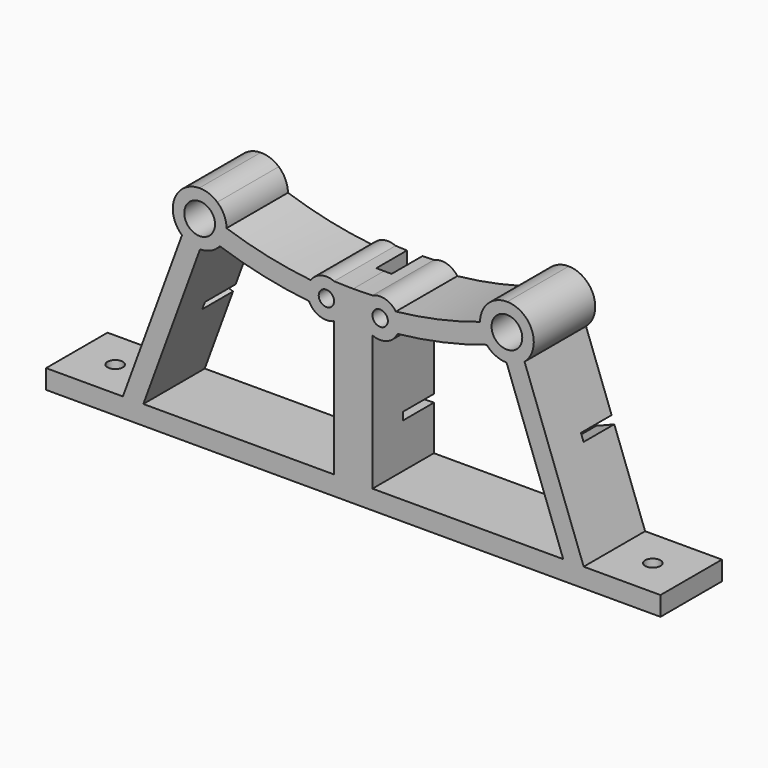
from build123d import *

# Parameters (mm, degrees)
F1_W      = 80
F1_H      = 5
F2_DEPTH  = 10
F3_W      = 5
F3_H      = 151.5
F4_DEPTH  = 10
F5_W      = 21
F5_H      = 23
F6_DEPTH  = 10
F8_DEPTH  = 10
F10_DEPTH = 10
F12_DEPTH = 10
F14_DEPTH = 20
F15_W     = 0.9078182304
F15_H     = 2
F16_DEPTH = 10
F17_R     = 135
F17_R_2   = 133
F18_DEPTH = 10
F19_R     = 7
F19_R_2   = 4
F20_DEPTH = 20
F21_R     = 4
F22_DEPTH = 20.001
F23_R     = 5
F23_R_2   = 2
F24_DEPTH = 20
F26_DEPTH = 20
F28_DEPTH = 20.001
F29_R     = 2
F30_DEPTH = 5.001


# Not quite as in the source:
# - ends of sketch curves that miss each other by under 0.0002 mm in the source are joined


with BuildPart() as f2:
    # F1 (on Front) → F2 (new body)
    with BuildSketch(Plane.XZ):
        with Locations((40, 2.5)):
            Rectangle(F1_W, F1_H)
    extrude(amount=F2_DEPTH)

    # F3 (on Front) → F4 (join, through all)
    with BuildSketch(Plane.XZ):
        with Locations((2.5, 75.75)):
            Rectangle(F3_W, F3_H)
    extrude(amount=F4_DEPTH)

    # F5 (on Front) → F6 (join, through all)
    with BuildSketch(Plane.XZ):
        with Locations((10.5, 151.5)):
            Rectangle(F5_W, F5_H)
    extrude(amount=F6_DEPTH)

    # F7 (on Front) → F8 (join, through all)
    with BuildSketch(Plane.XZ):
        Polygon((60, 5), (9.8688664765, 141.7212732458), (5.1744848971, 140), (55.3056184206, 3.2787267542), align=None)
    extrude(amount=F8_DEPTH)

    # F9 (on face) → F10 (join)
    with BuildSketch(Plane.XZ.offset(10)):
        Polygon((0, 163), (0, 0), (80, 0), (80, 5), (60, 5), (10.5, 140), (21, 140), (21, 163), align=None)
        Polygon((5.1744848971, 140), (54.6744848971, 5), (5, 5), (5, 140), align=None, mode=Mode.SUBTRACT)
    extrude(amount=F10_DEPTH)

    # F11 (on face) → F12 (cut)
    with BuildSketch(Plane(origin=(0, 0, 0), x_dir=(-1, 0, 0), z_dir=(0, 1, 0))):
        Polygon((-2, 0), (0, 0), (0, 140), (-21, 140), (-21, 138), (-2, 138), align=None)
    extrude(amount=-F12_DEPTH, mode=Mode.SUBTRACT)

    # F13 (on face) → F14 (join)
    with BuildSketch(Plane(origin=(0, 0, 0), x_dir=(-1, 0, 0), z_dir=(0, 1, 0))):
        Polygon((-2, 133), (-2, 138), (-11.2333333333, 138), (-13.0666666667, 133), align=None)
    extrude(amount=-F14_DEPTH)

    # F15 (on face) → F16 (join)
    with BuildSketch(Plane.XZ.offset(20)):
        with Locations((5.4539091152, 139)):
            Rectangle(F15_W, F15_H)
    extrude(amount=-F16_DEPTH)

    # F17 (on Front) → F18 (cut)
    with BuildSketch(Plane.XZ):
        with Locations((0, 151.5)):
            Circle(F17_R)
        with Locations((0, 151.5)):
            Circle(F17_R_2, mode=Mode.SUBTRACT)
    extrude(amount=F18_DEPTH, mode=Mode.SUBTRACT)

    # F19 (on Front) → F20 (join, through all)
    with BuildSketch(Plane.XZ):
        with Locations((40.0081513066, 52.2611576598)):
            Circle(F19_R)
        with Locations((40.0081513066, 52.2611576598)):
            Circle(F19_R_2, mode=Mode.SUBTRACT)
    extrude(amount=F20_DEPTH)

    # F21 (on Front) → F22 (cut, through all)
    with BuildSketch(Plane.XZ):
        with Locations((40.0081513066, 52.2611576598)):
            Circle(F21_R)
    extrude(amount=F22_DEPTH, mode=Mode.SUBTRACT)

    # F23 (on Front) → F24 (join, through all)
    with BuildSketch(Plane.XZ):
        with Locations((7, 44.7292174797)):
            Circle(F23_R)
        with Locations((7, 44.7292174797)):
            Circle(F23_R_2, mode=Mode.SUBTRACT)
    extrude(amount=F24_DEPTH)

    # F25 (on Front) → F26 (join, through all)
    with BuildSketch(Plane.XZ):
        with BuildLine():
            Line((8.7843409429, 47.3698633718), (8.9944926401, 44.8787117779))
            ThreePointArc((8.9944926401, 44.8787117779), (22.8274604253, 46.9633698145), (36.2703225327, 50.8348933176))
            Line((36.2703225327, 50.8348933176), (35.4228850903, 53.1868817915))
            ThreePointArc((35.4228850903, 53.1868817915), (22.294150224, 49.4058235462), (8.7843409429, 47.3698633718))
        make_face()
        with BuildLine():
            ThreePointArc((36.2703225327, 50.8348933176), (22.8274604253, 46.9633698145), (8.9944055882, 44.8787044343))
            Line((8.9944055882, 44.8787044343), (9.2046443373, 42.3875601839))
            ThreePointArc((9.2046443373, 42.3875601839), (23.3608559764, 44.5209347206), (37.117759975, 48.4829048437))
            Line((37.117759975, 48.4829048437), (36.2703225327, 50.8348933176))
        make_face()
    extrude(amount=F26_DEPTH)

    # F27 (on Front) → F28 (cut, through all)
    with BuildSketch(Plane.XZ):
        with BuildLine():
            ThreePointArc((5, 49.3117931746), (8.3573933592, 49.5414397593), (11.0998968806, 47.5911828128))
            ThreePointArc((11.0998968806, 47.5911828128), (22.1823046987, 49.3814641789), (33.0087181874, 52.3502419386))
            ThreePointArc((33.0087181874, 52.3502419386), (38.6064619078, 59.1193838757), (46.4113234148, 55.0894764101))
            ThreePointArc((46.4113234148, 55.0894764101), (104.3190443402, 175.3020374745), (0, 258.5))
            Line((0, 258.5), (0, 253.8104570129))
            ThreePointArc((0, 253.8104570129), (-102.2798898997, 148.9992528562), (5, 49.3117931746))
        make_face()
    extrude(amount=F28_DEPTH, mode=Mode.SUBTRACT)

    # F29 (on face) → F30 (cut, through all)
    with BuildSketch(Plane.XY.offset(5)):
        with Locations((70, -10)):
            Circle(F29_R)
    extrude(amount=-F30_DEPTH, mode=Mode.SUBTRACT)

    # F31: F2 across plane


with BuildPart() as f2_1:
    add(f2.part)
    add(f2.part.mirror(Plane.YZ))


solid = f2_1.part
